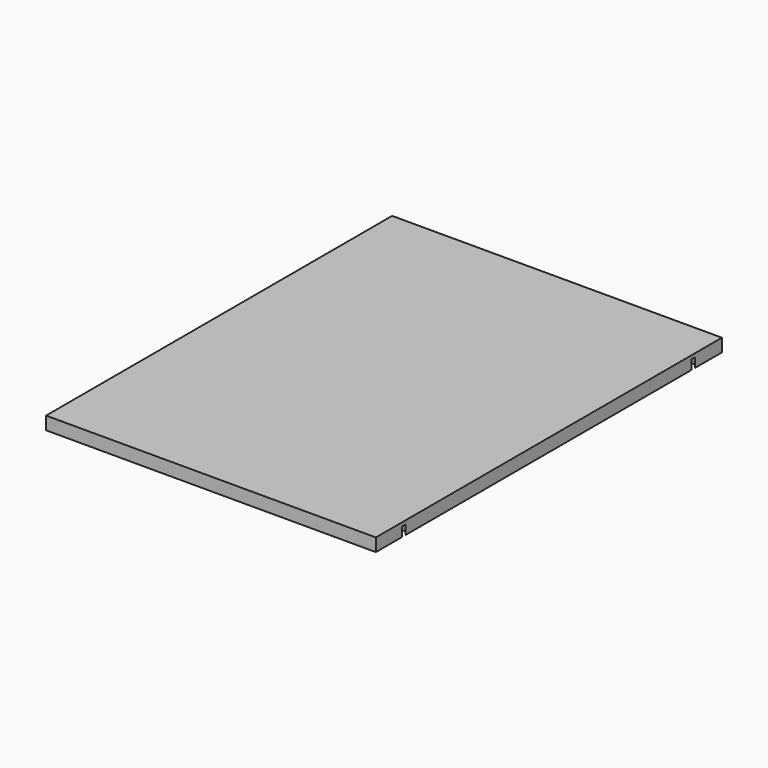
from build123d import *

# Parameters (mm, degrees)
F0_W     = 457.5
F0_H     = 600
F1_DEPTH = 9
F2_R     = 10
F3_DEPTH = 13


with BuildPart() as f1:
    # F0 (on Top) → F1 (new body, symmetric)
    with BuildSketch(Plane.XY):
        Rectangle(F0_W, F0_H)
    extrude(amount=F1_DEPTH, both=True)

    # F2 (on face) → F3 (cut)
    with BuildSketch(Plane(origin=(0, 0, -9), x_dir=(1, 0, 0), z_dir=(0, 0, -1))):
        with Locations((-219.25, 252)):
            Circle(F2_R)
        with Locations((-219.25, -250)):
            Circle(F2_R)
        with Locations((219.25, 252)):
            Circle(F2_R)
        with Locations((219.25, -250)):
            Circle(F2_R)
    extrude(amount=-F3_DEPTH, mode=Mode.SUBTRACT)


solid = f1.part
